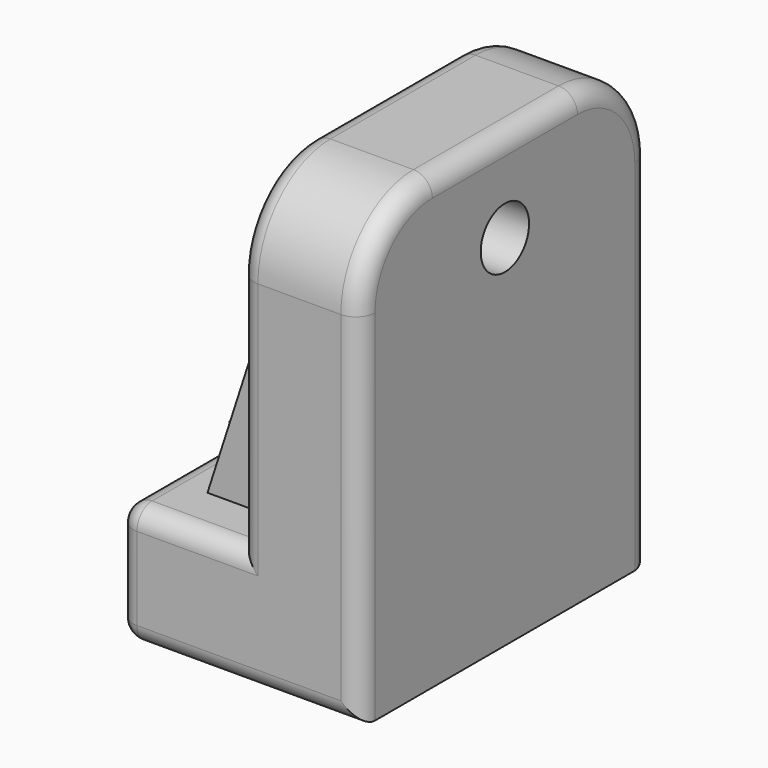
from build123d import *

# Parameters (mm, degrees)
F1_DEPTH  = 76.2
F2_R      = 12.7
F3_DEPTH  = 101.601
F5_DEPTH  = 50.801
F6_R      = 38.1
F7_R      = 17.78
F7_R_2    = 12.7
F8_DEPTH  = 6.35
F12_DEPTH = 6.35
F15_DEPTH = 6.35
F16_R     = 7.971733183


# Not quite as in the source:
# - a pattern or mirror of a feature is missing from the dataset's text; its kind, count and spacing are read off the source's solid


with BuildPart() as f1:
    # F0 (on Front) → F1 (new body, symmetric)
    with BuildSketch(Plane.XZ):
        Polygon((-101.6, 0), (0, 0), (0, 188.9744497656), (-50.8, 188.9744497656), (-50.8, 50.8), (-101.6, 50.8), align=None)
    extrude(amount=F1_DEPTH, both=True)

    # F2 (on face) → F3 (cut, through all)
    with BuildSketch(Plane.YZ):
        with Locations((0, 150.8744497656)):
            Circle(F2_R)
    extrude(amount=-F3_DEPTH, mode=Mode.SUBTRACT)

    # F4 (on face) → F5 (cut, through all)
    with BuildSketch(Plane.XY.offset(50.8)):
        with BuildLine():
            Line((-88.9, 12.7), (-101.6, 12.7))
            Line((-101.6, 12.7), (-101.6, -12.7))
            Line((-101.6, -12.7), (-88.9, -12.7))
            ThreePointArc((-88.9, -12.7), (-76.2, 0), (-88.9, 12.7))
        make_face()
    extrude(amount=-F5_DEPTH, mode=Mode.SUBTRACT)

    # F6
    f6_edges = [f1.edges().sort_by_distance(p)[0] for p in [
        (-25.4, -76.2, 188.97445),
        (-25.4, 76.2, 188.97445),
    ]]
    fillet(f6_edges, radius=F6_R)

    # F7 (on face) → F8 (cut)
    with BuildSketch(Plane(origin=(-50.8, 0, 0), x_dir=(0, -1, 0), z_dir=(-1, 0, 0))):
        with Locations((0, 150.8744497656)):
            Circle(F7_R)
        with Locations((0, 150.8744497656)):
            Circle(F7_R_2, mode=Mode.SUBTRACT)
    extrude(amount=-F8_DEPTH, mode=Mode.SUBTRACT)

    # F11 (on offset) → F12 (join, symmetric)
    with BuildSketch(Plane.XZ.offset(45.974)):
        Polygon((-83.1002444029, 50.8), (-50.8, 50.8), (-50.8, 150.8744497656), align=None)
    f12 = extrude(amount=F12_DEPTH, both=True)

    # F12_copies: F12 across plane
    add(f12.mirror(Plane.ZX))

    # F14 (on face) → F15 (join)
    with BuildSketch(Plane.XY.offset(50.8)):
        with BuildLine():
            Line((-101.6, -12.7), (-101.6, -17.5260007381))
            Line((-101.6, -17.5260007381), (-88.9, -17.5260007381))
            ThreePointArc((-88.9, -17.5260007381), (-71.3739992619, 0), (-88.9, 17.5260007381))
            Line((-88.9, 17.5260007381), (-101.6, 17.5260007381))
            Line((-101.6, 17.5260007381), (-101.6, 12.7))
            Line((-101.6, 12.7), (-88.9, 12.7))
            ThreePointArc((-88.9, 12.7), (-76.2, 0), (-88.9, -12.7))
            Line((-88.9, -12.7), (-101.6, -12.7))
        make_face()
    extrude(amount=F15_DEPTH)

    # F16
    f16_edges = [f1.edges().sort_by_distance(p)[0] for p in [
        (-76.2, -76.2, 50.8),
        (-76.2, 76.2, 50.8),
        (-50.8, -76.2, 0),
        (0, -76.2, 75.437225),
        (-25.4, -76.2, 150.87445),
        (-50.8, -76.2, 100.837225),
        (-101.6, -76.2, 25.4),
        (-50.8, 76.2, 0),
        (-101.6, 76.2, 25.4),
        (-101.6, 46.863, 50.8),
        (-101.6, -46.863, 50.8),
        (-101.6, -44.45, 0),
        (-101.6, 44.45, 0),
        (0, 76.2, 75.437225),
        (-50.8, 76.2, 100.837225),
        (0, 65.040768, 177.815218),
        (-50.8, 65.040768, 177.815218),
        (0, 0, 188.97445),
        (-50.8, 0, 188.97445),
        (-50.8, -65.040768, 177.815218),
        (0, -65.040768, 177.815218),
    ]]
    fillet(f16_edges, radius=F16_R)


solid = f1.part
